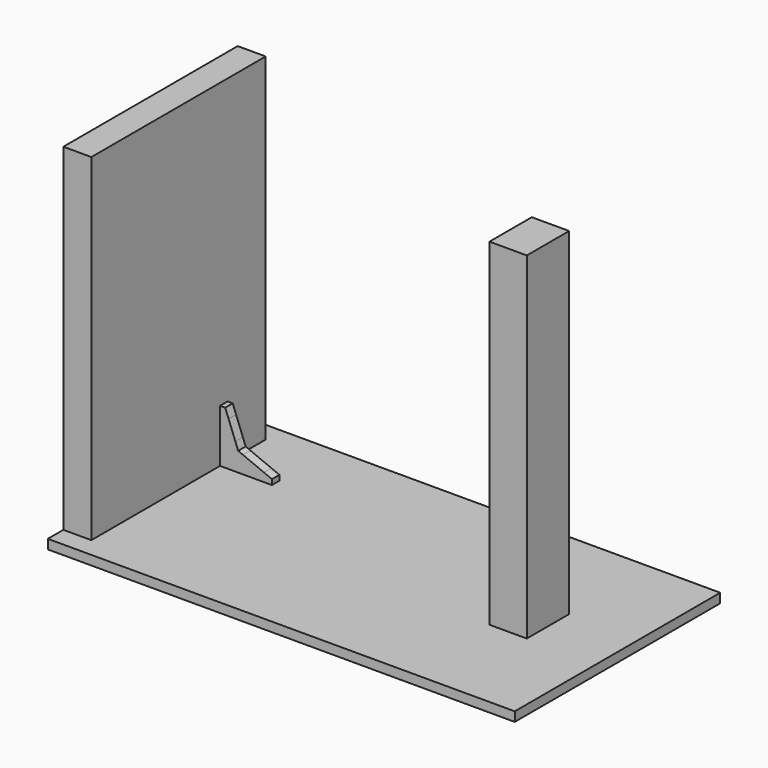
from build123d import *

# Parameters (mm, degrees)
F0_W      = 900
F0_H      = 495
F1_DEPTH  = 18
F2_W      = 54
F2_H      = 420
F3_DEPTH  = 650
F2_W_2    = 72
F2_H_2    = 102
F4_W      = 102
F4_H      = 650
F5_DEPTH  = 766.001
F6_W      = 18
F6_H      = 102
F7_DEPTH  = 100
F8_DEPTH  = 650
F10_DEPTH = 25


# Not quite as in the source:
# - a feature names something its author has since deleted; it is built from what else it names


with BuildPart() as f1:
    # F0 (on Top) → F1 (new body)
    with BuildSketch(Plane.XY):
        Rectangle(F0_W, F0_H)
    extrude(amount=F1_DEPTH)


with BuildPart() as f3:
    # F2 (on face) → F3 (new body)
    with BuildSketch(Plane.XY.offset(18)):
        with Locations((-423, 0)):
            Rectangle(F2_W, F2_H)
    extrude(amount=F3_DEPTH)


with BuildPart() as f3b:
    # F2 (on face) → F3, piece 2 (new body)
    with BuildSketch(Plane.XY.offset(18)):
        with Locations((280, 0)):
            Rectangle(F2_W_2, F2_H_2)
    extrude(amount=F3_DEPTH)


with BuildPart() as f5_tool:
    # F4 (on face) → F5 (new body, through all)
    with BuildSketch(Plane.YZ.offset(316)):
        with Locations((0, 343)):
            Rectangle(F4_W, F4_H)
    extrude(amount=-F5_DEPTH)


with BuildPart() as f3_1:
    add(f3.part)

    # F5: cut by f5_tool
    add(f5_tool.part, mode=Mode.SUBTRACT)

    # F2 (on face) → F8 (join)
    with BuildSketch(Plane.XY.offset(18)):
        with Locations((-423, 0)):
            Rectangle(F2_W, F2_H)
    extrude(amount=F8_DEPTH)


with BuildPart() as f3b_1:
    add(f3b.part)

    # F5: cut by f5_tool
    add(f5_tool.part, mode=Mode.SUBTRACT)


with BuildPart() as f7:
    # F6 (on face) → F7 (new body)
    with BuildSketch(Plane.YZ.offset(-396)):
        with Locations((109, 69)):
            Rectangle(F6_W, F6_H)
    extrude(amount=F7_DEPTH)

    # F9 (on face) → F10 (cut)
    with BuildSketch(Plane(origin=(0, 118, 0), x_dir=(-1, 0, 0), z_dir=(0, 1, 0))):
        Polygon((361, 55), (366.4967978412, 69.2916743872), (379.5285465821, 103.1742211134), (386, 120), (296, 120), (296, 28), (311.3627376398, 34.3814448658), (351.799326006, 51.1781815717), align=None)
    extrude(amount=-F10_DEPTH, mode=Mode.SUBTRACT)


with BuildPart() as f8:
    # F2 (on face) → F8, piece 2 (new body)
    with BuildSketch(Plane.XY.offset(18)):
        with Locations((280, 0)):
            Rectangle(F2_W_2, F2_H_2)
    extrude(amount=F8_DEPTH)


solid = Compound([f1.part, f3_1.part, f7.part, f8.part])
